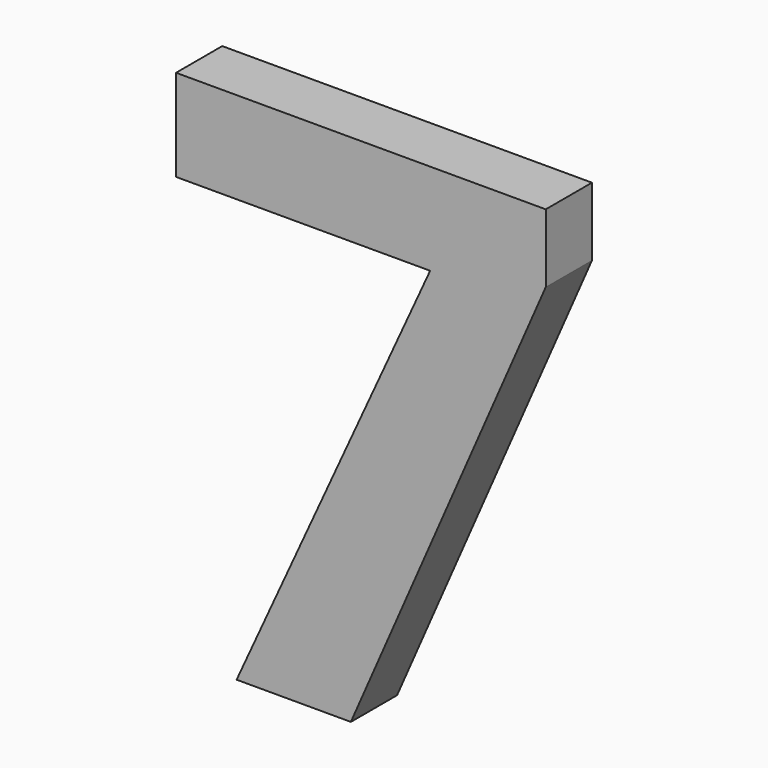
from build123d import *

# Parameters (mm, degrees)
F0_TEXT_SIZE = 62.5
F1_DEPTH     = 5


# Not quite as in the source:
# - Text() gives the source's letters only with a copy of the font that has no kerning and outlines rounded to 1/6400 em; it was checked with that copy


with BuildPart() as f1:
    # F0 (on Front) → F1 (new body)
    with BuildSketch(Plane.XZ):
        with Locations((-53.576233034, 13.2174881031)):
            Text('7', F0_TEXT_SIZE, font='Open Sans', font_style=FontStyle.BOLD, text_align=(TextAlign.LEFT, TextAlign.BOTTOM))
    extrude(amount=F1_DEPTH)


solid = f1.part
